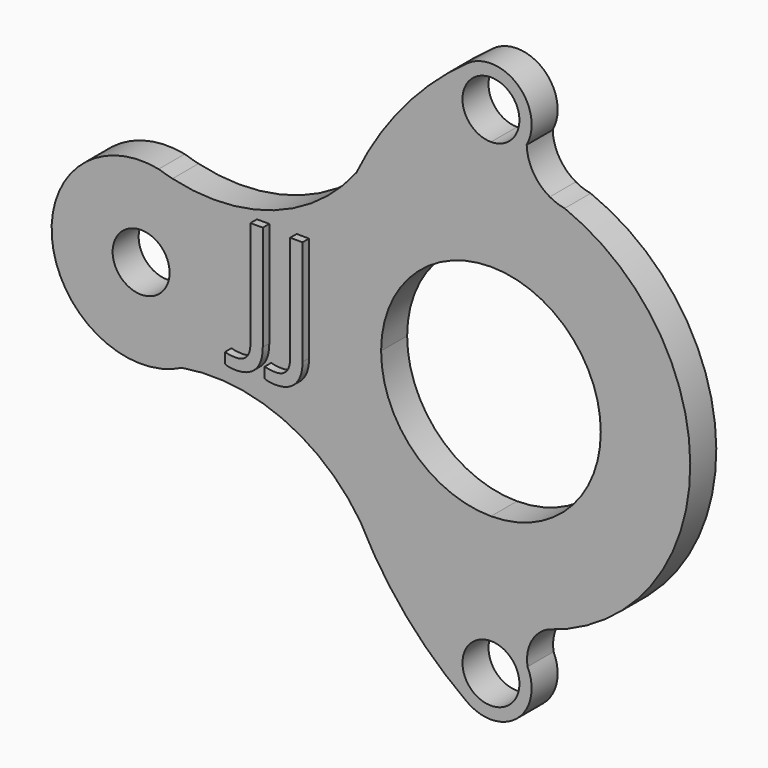
from build123d import *

# Parameters (mm, degrees)
F0_R         = 7
F1_DEPTH     = 8
F2_TEXT_SIZE = 36.5894805226
F3_DEPTH     = 2


# Not quite as in the source:
# - Text() gives the source's letters only with a copy of the font that has no kerning and outlines rounded to 1/6400 em; it was checked with that copy


with BuildPart() as f1:
    # F0 (on Front) → F1 (new body)
    with BuildSketch(Plane.XZ):
        with BuildLine():
            ThreePointArc((-33.0814872484, 36.6005988435), (-53.3026603657, 21.8775923368), (-78.2833795427, 20.6022758141))
            ThreePointArc((-78.2833795427, 20.6022758141), (-79.9853244925, 21.0517972552), (-81.6678607395, 21.5692505532))
            ThreePointArc((-81.6678607395, 21.5692505532), (-107.792813133, -3.0121911879), (-75.9794818803, -19.5854337867))
            ThreePointArc((-75.9794818803, -19.5854337867), (-51.2108921595, -22.5558287126), (-32.100327298, -38.5899359046))
            ThreePointArc((-32.100327298, -38.5899359046), (-20.795221141, -55.4415559973), (-5.8179797945, -69.1333333333))
            ThreePointArc((-5.8179797945, -69.1333333333), (6.4398042277, -68.6504196949), (9.0065538889, -56.6546591566))
            ThreePointArc((9.0065538889, -56.6546591566), (9.8398737977, -51.0307376995), (13.8509787315, -47.001599847))
            ThreePointArc((13.8509787315, -47.001599847), (48.9478289237, -2.2605405675), (18.1240981854, 45.5249059852))
            ThreePointArc((18.1240981854, 45.5249059852), (16.2405247742, 46.0102550599), (14.4696355434, 46.8148443043))
            ThreePointArc((14.4696355434, 46.8148443043), (10.39126819, 50.7756642661), (8.789283796, 56.2304622496))
            ThreePointArc((8.789283796, 56.2304622496), (6.620285675, 68.4947860264), (-5.8179797945, 69.1333333333))
            ThreePointArc((-5.8179797945, 69.1333333333), (-21.5131306884, 54.5961611569), (-33.0814872484, 36.6005988435))
        make_face()
        with BuildLine():
            ThreePointArc((7, -61), (-4.9497474683, -65.9497474683), (0, -54))
            ThreePointArc((0, -54), (4.9497474683, -56.0502525317), (7, -61))
        make_face(mode=Mode.SUBTRACT)
        with Locations((-86, 0)):
            Circle(F0_R, mode=Mode.SUBTRACT)
        with BuildLine():
            ThreePointArc((0, 27), (19.091883092, 19.091883092), (27, 0))
            ThreePointArc((27, 0), (19.091883092, -19.091883092), (0, -27))
            ThreePointArc((0, -27), (-19.091883092, -19.091883092), (-27, 0))
            ThreePointArc((-27, 0), (-19.091883092, 19.091883092), (0, 27))
        make_face(mode=Mode.SUBTRACT)
        with BuildLine():
            ThreePointArc((7, 61), (4.9497474683, 56.0502525317), (0, 54))
            ThreePointArc((0, 54), (-4.9497474683, 65.9497474683), (7, 61))
        make_face(mode=Mode.SUBTRACT)
    extrude(amount=F1_DEPTH)

    # F2 (on face) → F3 (join)
    with BuildSketch(Plane.XZ.offset(8)):
        with Locations((-60.9240047634, -7.5678899884)):
            Text('JJ', F2_TEXT_SIZE, font='Open Sans', text_align=(TextAlign.LEFT, TextAlign.BOTTOM))
    extrude(amount=F3_DEPTH)


solid = f1.part
